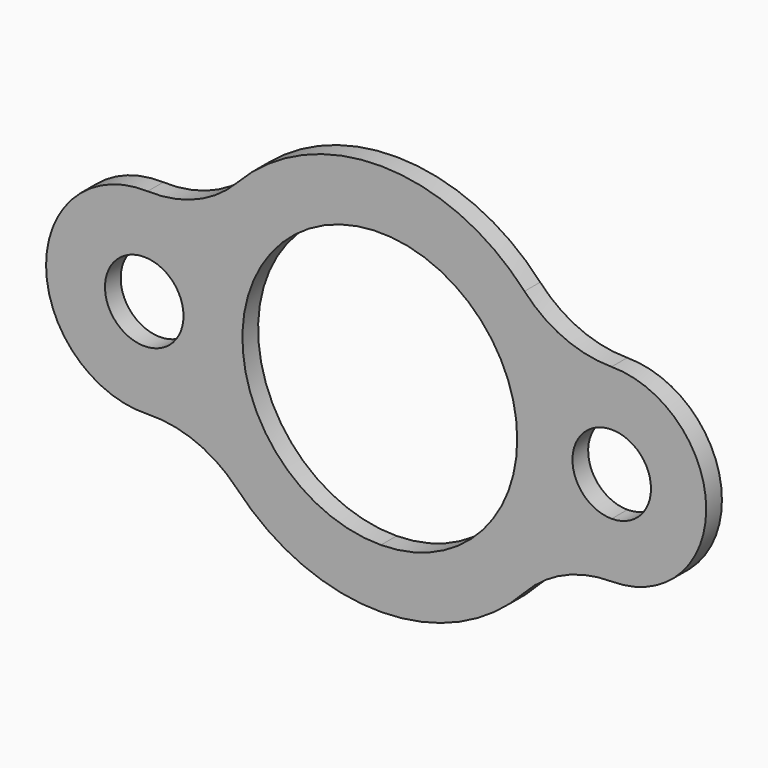
from build123d import *

# Parameters (mm, degrees)
F0_R     = 12.7
F1_DEPTH = 6.35


# Not quite as in the source:
# - a length typed as a fraction of an inch, garbled in the dataset ("3 / 203.2 mm" for 3/8 in), is restored


with BuildPart() as f1:
    # F0 (on Front) → F1 (new body)
    with BuildSketch(Plane.XZ):
        with BuildLine():
            ThreePointArc((-46.13671875, -43.6308741946), (-24.8918341596, -58.4178619274), (0.4890866537, -63.4981164622))
            ThreePointArc((0.4890866537, -63.4981164622), (25.7887406506, -58.0275008566), (46.8033281156, -42.9150145905))
            ThreePointArc((46.8033281156, -42.9150145905), (59.5789989506, -33.7738186545), (74.9568035052, -30.5640903944))
            ThreePointArc((74.9568035052, -30.5640903944), (105.5782883644, 0), (74.9568035052, 30.5640903944))
            ThreePointArc((74.9568035052, 30.5640903944), (59.5789989506, 33.7738186545), (46.8033281156, 42.9150145905))
            ThreePointArc((46.8033281156, 42.9150145905), (0.4890866537, 63.4981164622), (-46.13671875, 43.6308741946))
            ThreePointArc((-46.13671875, 43.6308741946), (-59.3475236203, 34.5646316236), (-75.1176136364, 31.7315448688))
            ThreePointArc((-75.1176136364, 31.7315448688), (-107.95, 0), (-75.1176136364, -31.7315448688))
            ThreePointArc((-75.1176136364, -31.7315448688), (-59.3475236203, -34.5646316236), (-46.13671875, -43.6308741946))
        make_face()
        with Locations((-76.2, 0)):
            Circle(F0_R, mode=Mode.SUBTRACT)
        with BuildLine():
            ThreePointArc((0.3423606576, -44.4486815235), (-31.5517070159, 31.3096196781), (44.45, 0))
            ThreePointArc((44.45, 0), (31.5517070159, -31.3096196781), (0.3423606576, -44.4486815235))
        make_face(mode=Mode.SUBTRACT)
        with BuildLine():
            ThreePointArc((87.7141441822, 0), (83.9859725242, -8.9886759982), (74.9903180088, -12.6999776501))
            ThreePointArc((74.9903180088, -12.6999776501), (66.0423158402, 8.9886759982), (87.7141441822, 0))
        make_face(mode=Mode.SUBTRACT)
    extrude(amount=F1_DEPTH)


solid = f1.part
